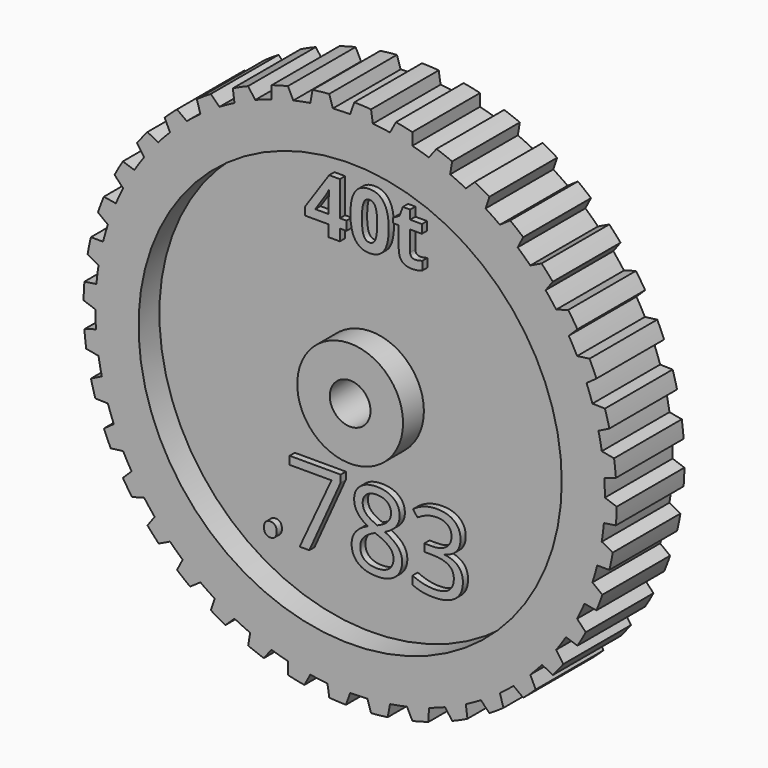
from build123d import *

# Parameters (mm, degrees)
F0_R            = 19.8755
F0_R_2          = 1.5875
F1_DEPTH        = 6.604
F2_R            = 16.5735
F2_R_2          = 4.1275
F3_DEPTH        = 2.032
F4_R            = 16.51
F4_R_2          = 4.1275
F5_DEPTH        = 2.032
F8_DEPTH        = 6.604
F9_COUNT        = 40
F9_ANGLE        = 351
F10_TEXT_SIZE   = 5.9922109358
F10_TEXT_SIZE_2 = 8.3916128561
F11_DEPTH       = 0.508


# Not quite as in the source:
# - Text() gives the source's letters only with a copy of the font that has no kerning and outlines rounded to 1/6400 em; it was checked with that copy


with BuildPart() as f1:
    # F0 (on Front) → F1 (new body)
    with BuildSketch(Plane.XZ):
        Circle(F0_R)
        Circle(F0_R_2, mode=Mode.SUBTRACT)
    extrude(amount=F1_DEPTH)

    # F2 (on Front) → F3 (cut)
    with BuildSketch(Plane.XZ):
        Circle(F2_R)
        Circle(F2_R_2, mode=Mode.SUBTRACT)
    extrude(amount=F3_DEPTH, mode=Mode.SUBTRACT)

    # F4 (on face) → F5 (cut)
    with BuildSketch(Plane.XZ.offset(6.604)):
        Circle(F4_R)
        Circle(F4_R_2, mode=Mode.SUBTRACT)
    extrude(amount=-F5_DEPTH, mode=Mode.SUBTRACT)

    # F7 (on Front) → F8 (join, through all)
    with BuildSketch(Plane.XZ):
        with BuildLine():
            Line((1.7713056339, 19.7964132257), (1.6291638932, 20.7349634501))
            ThreePointArc((1.6291638932, 20.7349634501), (0.9771726634, 20.7759679676), (0.3242142115, 20.7964422002))
            Line((0.3242142115, 20.7964422002), (0, 19.8755))
            ThreePointArc((0, 19.8755), (0.886535161, 19.8557184624), (1.7713056339, 19.7964132257))
        make_face()
    extrude(amount=F8_DEPTH)

    # F9: F1 ×40 about axis
    f9_axis = Axis((0, -4.5361137018, 0), (0, -1, 0))


with BuildPart() as f1_1:
    add(f1.part)
    for i in range(1, F9_COUNT):
        add(f1.part.rotate(f9_axis, i * F9_ANGLE / (F9_COUNT - 1)))

    # F10 (on face) → F11 (join)
    with BuildSketch(Plane.XZ.offset(4.572)):
        with Locations((-4.8346826807, 9.8623242229)):
            Text('40t', F10_TEXT_SIZE, font='Open Sans', font_style=FontStyle.BOLD, text_align=(TextAlign.LEFT, TextAlign.BOTTOM))
        with Locations((-8.5594709963, -12.1277468279)):
            Text('.783', F10_TEXT_SIZE_2, font='Open Sans', text_align=(TextAlign.LEFT, TextAlign.BOTTOM))
    extrude(amount=F11_DEPTH)


solid = f1_1.part
